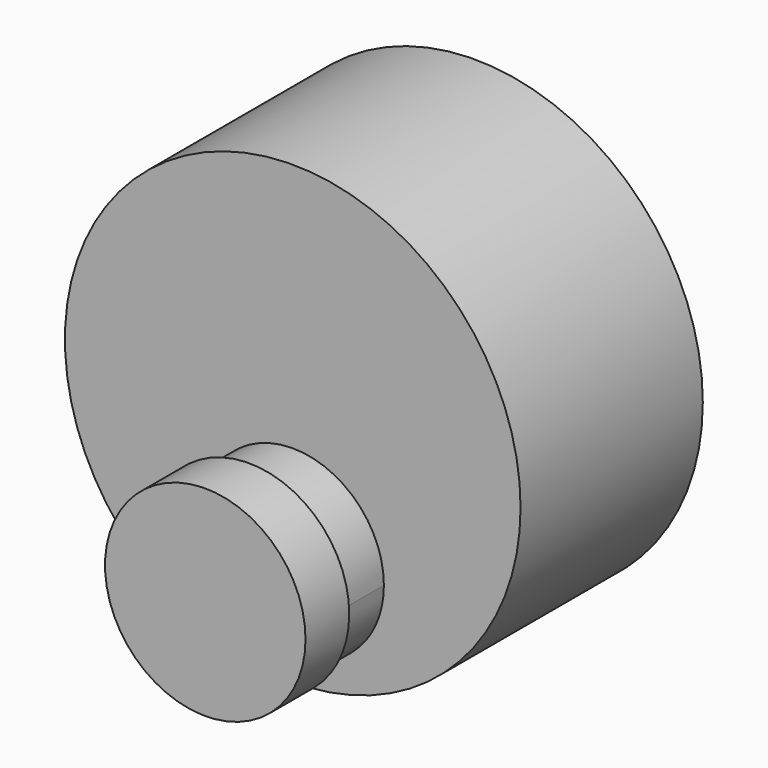
from build123d import *

# Parameters (mm, degrees)
F0_R     = 25
F0_R_2   = 20
F1_DEPTH = 20
F2_R     = 25
F2_R_2   = 10
F3_DEPTH = 5
F2_R_3   = 7.5
F4_DEPTH = 15
F5_R     = 11
F5_R_2   = 10
F5_R_3   = 7.5
F6_DEPTH = 2
F7_DEPTH = 4


with BuildPart() as f1:
    # F0 (on Front) → F1 (new body)
    with BuildSketch(Plane.XZ):
        Circle(F0_R)
        Circle(F0_R_2, mode=Mode.SUBTRACT)
    extrude(amount=F1_DEPTH)

    # F2 (on face) → F3 (join)
    with BuildSketch(Plane.XZ.offset(20)):
        Circle(F2_R)
        with Locations((0, -12.3999994248)):
            Circle(F2_R_2, mode=Mode.SUBTRACT)
    extrude(amount=F3_DEPTH)

    # F2 (on face) → F4 (join)
    with BuildSketch(Plane.XZ.offset(20)):
        with BuildLine():
            ThreePointArc((8.0763880603, -18.2967744671), (9.5069416902, -15.5012991037), (10, -12.3999994248))
            ThreePointArc((10, -12.3999994248), (-3.1012996789, -2.8930577346), (-8.0763880603, -18.2967744671))
            ThreePointArc((-8.0763880603, -18.2967744671), (0, -20), (8.0763880603, -18.2967744671))
        make_face()
        with Locations((0, -12.3999994248)):
            Circle(F2_R_3, mode=Mode.SUBTRACT)
        with BuildLine():
            ThreePointArc((8.0763880603, -18.2967744671), (0, -20), (-8.0763880603, -18.2967744671))
            ThreePointArc((-8.0763880603, -18.2967744671), (0, -22.3999994248), (8.0763880603, -18.2967744671))
        make_face()
    extrude(amount=F4_DEPTH)


with BuildPart() as f6:
    # F5 (on face) → F6 (new body)
    with BuildSketch(Plane.XZ.offset(35)):
        with Locations((0, -12.3999994248)):
            Circle(F5_R)
        with Locations((0, -12.3999994248)):
            Circle(F5_R_2, mode=Mode.SUBTRACT)
        with Locations((0, -12.3999994248)):
            Circle(F5_R_2)
        with Locations((0, -12.3999994248)):
            Circle(F5_R_3, mode=Mode.SUBTRACT)
        with Locations((0, -12.3999994248)):
            Circle(F5_R_3)
    extrude(amount=F6_DEPTH)

    # F7 (add): a face of the model
    f7_faces = [f6.faces().sort_by_distance(p)[0] for p in [
        (0, -35, -12.3999994248),
    ]]
    extrude(f7_faces, amount=F7_DEPTH)


solid = Compound([f1.part, f6.part])
